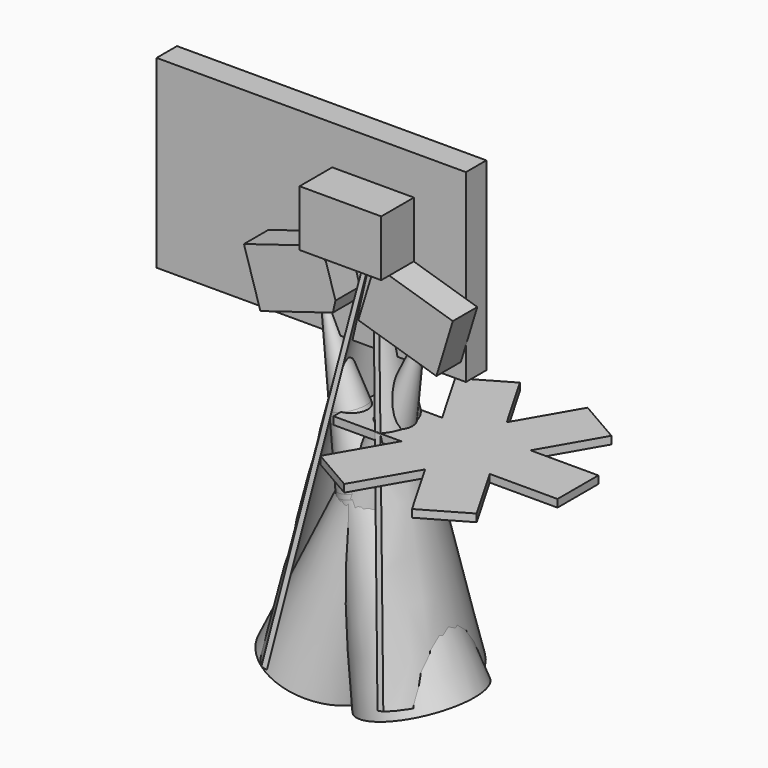
from build123d import *

# Parameters (mm, degrees)
F3_DEPTH  = 0.3
F6_DEPTH  = 1.2
F7_DEPTH  = 1.6
F8_W      = 12.1187474579
F8_H      = 7.2388057597
F9_DEPTH  = 1
F13_DEPTH = 12.5


# Not quite as in the source:
# - a feature names something its author has since deleted; it is built from what else it names


with BuildPart() as f2:
    # F1 (on Front) → F2 (revolve)
    with BuildSketch(Plane.XZ):
        Polygon((-3.7210601673, -9.810751838), (-4.7051198674, -2.8088032427), (-4.7835134136, -2.9695338315), (-3.8178826888, -9.8403534535), align=None)
        Polygon((-5.1072294295, -0.6661746932), (-5.044458455, -0.3942837314), (-5.1027113349, 0.0202070469), (-5.1654823095, -0.2516839149), align=None)
        Polygon((-4.7051198674, -2.8088032427), (-4.7300080769, -2.6317144309), (-4.808401623, -2.7924450197), (-4.7835134136, -2.9695338315), align=None)
        Polygon((-5.1654823095, -0.2516839149), (-5.1027113349, 0.0202070469), (-5.5609535977, 3.280770169), (-5.6599804046, 3.2668528589), align=None)
        Polygon((-4.808401623, -2.7924450197), (-4.7300080769, -2.6317144309), (-5.044458455, -0.3942837314), (-5.1072294295, -0.6661746932), align=None)
    revolve(axis=Axis((-5.5178402688, 0, 3.1482272372), (0.2923717047, 0, -0.956304756)))


with BuildPart() as f3:
    # F0 (on Top) → F3 (new body)
    with BuildSketch(Plane.XY):
        Polygon((-3.0597665006, 3.2996710384), (-1.7320508076, 1), (-4.295240622, 1), (-4.295240622, 0), (-4.3874821937, 0), (-4.3874821937, -1), (-1.7320508076, -1), (-3.0597665006, -3.2996710384), (-1.3277156931, -4.2996710384), (0, -2), (1.3277156931, -4.2996710384), (3.0597665006, -3.2996710384), (1.7320508076, -1), (4.3874821937, -1), (4.3874821937, 1), (1.7320508076, 1), (3.0597665006, 3.2996710384), (1.3277156931, 4.2996710384), (0, 2), (-1.3277156931, 4.2996710384), align=None)
    extrude(amount=-F3_DEPTH)


with BuildPart() as f5:
    # F4 (on Front) → F5 (revolve)
    with BuildSketch(Plane.XZ):
        Polygon((-3.6452723001, 5.6662573418), (-3.7914278099, 5.7), (-7.0850528365, -8.5662573418), (-6.9388973268, -8.6), align=None)
    revolve(axis=Axis((-3.6374821937, 0, 5.545), (0, 0, -1)))

    # F12 (on Right) → F13 (cut, symmetric)
    with BuildSketch(Plane.YZ):
        Polygon((-2.7707505506, -10.2039054036), (0, 5.6963409297), (-10.1999649778, -10.2039054036), align=None)
    extrude(amount=F13_DEPTH, both=True, mode=Mode.SUBTRACT)


with BuildPart() as f6:
    # F1 (on Front) → F6 (new body)
    with BuildSketch(Plane.XZ):
        Polygon((-5.2261826705, 5.7), (-4.6248886842, 5.7), (-4.6762880239, 5.868119665), align=None)
        Polygon((-4.5701869432, 5.5210786674), (-4.6248886842, 5.7), (-5.2261826705, 5.7), (-7.736463243, 4.9325302099), (-7.0932454926, 2.8286597468), (-5.6599804046, 3.2668528589), (-5.5631578831, 3.2964544743), (-4.2539193968, 3.6967288489), (-4.1500189554, 4.1467711043), (-4.5301121729, 5.39), (-4.5701869432, 5.39), align=None)
    extrude(amount=F6_DEPTH)


with BuildPart() as f6b:
    # F1 (on Front) → F6, piece 2 (new body)
    with BuildSketch(Plane.XZ):
        Polygon((-2.0643619298, 5.7), (-2.6656559161, 5.7), (-3.2574743268, 3.7642492019), (-1.8242092387, 3.3260560898), (-1.7273867172, 3.2964544743), (-0.1972991077, 2.8286597468), (0.4459186427, 4.9325302099), align=None)
        Polygon((-2.6142565764, 5.868119665), (-2.6656559161, 5.7), (-2.0643619298, 5.7), align=None)
    extrude(amount=F6_DEPTH)


with BuildPart() as f7:
    # F1 (on Front) → F7 (new body)
    with BuildSketch(Plane.XZ):
        Polygon((-3.6374821937, 5.7), (-2.9229645152, 5.7), (-2.6656559161, 5.7), (-2.6142565764, 5.868119665), (-2.0643619298, 5.7), (-2.0374821937, 5.7), (-2.0374821937, 7.9), (-5.2374821937, 7.9), (-5.2374821937, 6.6), (-5.2374821937, 5.7), (-5.2261826705, 5.7), (-4.6762880239, 5.868119665), (-4.6248886842, 5.7), (-4.5701869432, 5.7), (-3.7914278099, 5.7), align=None)
        Polygon((-2.6142565764, 5.868119665), (-2.6656559161, 5.7), (-2.0643619298, 5.7), align=None)
        Polygon((-5.2261826705, 5.7), (-4.6248886842, 5.7), (-4.6762880239, 5.868119665), align=None)
    extrude(amount=F7_DEPTH)


with BuildPart() as f9:
    # F8 (on Front) → F9 (new body)
    with BuildSketch(Plane.XZ):
        with Locations((-6.0593737289, 5.8194028798)):
            Rectangle(F8_W, F8_H)
    extrude(amount=-F9_DEPTH)


with BuildPart() as f11:
    # F10 (on Front) → F11 (revolve)
    with BuildSketch(Plane.XZ):
        Polygon((-1.8150609466, 3.1166956651), (-1.9049403512, 3.1605327798), (-7.6195546574, -8.5561628853), (-7.5296752528, -8.6), align=None)
    revolve(axis=Axis((-1.7727043315, 0, 3.1482272372), (-0.2923717047, 0, -0.956304756)))


solid = Compound([f2.part, f3.part, f5.part, f6.part, f6b.part, f7.part, f9.part, f11.part])
